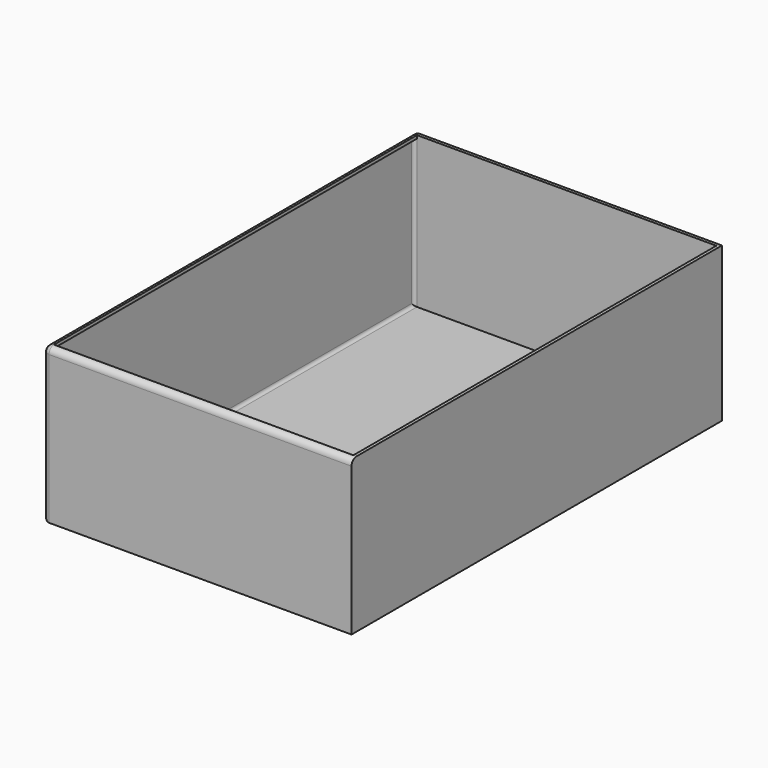
from build123d import *

# Parameters (mm, degrees)
F0_W     = 254
F0_H     = 381
F1_DEPTH = 127
F2_R     = 5.08
F3_T     = -2.54


# Not quite as in the source:
# - a shell that OpenCascade refuses in one call is made with other operations: the cavity is built on its own and cut out


with BuildPart() as f1:
    # F0 (on Top) → F1 (new body)
    with BuildSketch(Plane.XY):
        with Locations((-127, -190.5)):
            Rectangle(F0_W, F0_H)
    extrude(amount=F1_DEPTH)

    # F2
    f2_edges = [f1.edges().sort_by_distance(p)[0] for p in [
        (-254, -190.5, 127),
        (-127, -381, 127),
        (-254, 0, 63.5),
        (-254, -381, 63.5),
        (-254, -190.5, 0),
    ]]
    fillet(f2_edges, radius=F2_R)

    # F3: a shell. OpenCascade refuses it in one call, so the cavity is built on its own and cut out:
    # the body offset inwards by the wall thickness, plus a prism from it out through each open face.
    f3_core = offset(f1.part, amount=F3_T, mode=Mode.PRIVATE)
    f3_exits = [f3_core.faces().sort_by_distance(p)[0] for p in [
        (-125.73, -189.23, 124.46),
    ]]
    add(f3_core, mode=Mode.SUBTRACT)
    extrude(f3_exits, amount=-F3_T, mode=Mode.SUBTRACT)


solid = f1.part
